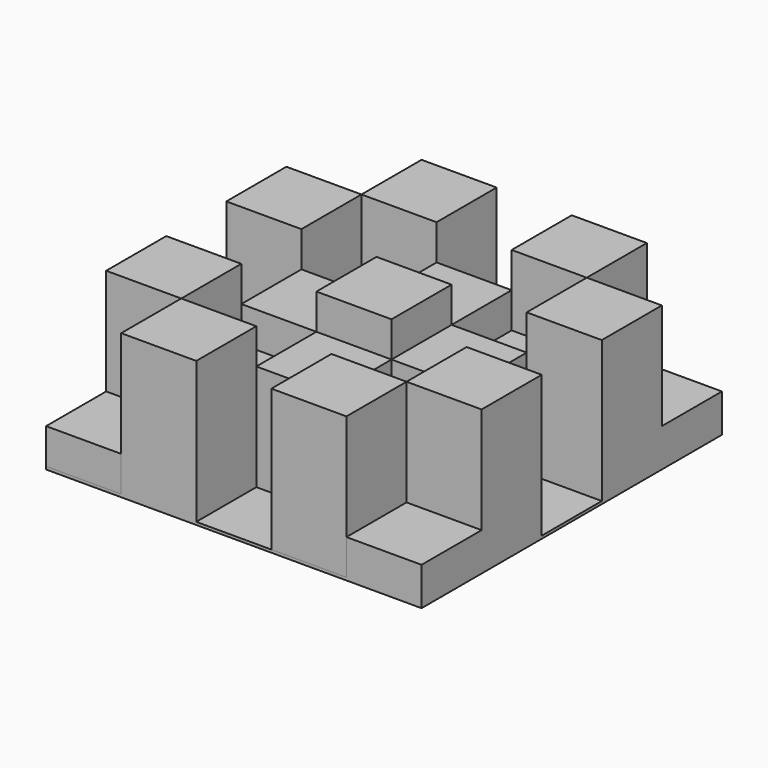
from build123d import *

# Parameters (mm, degrees)
F0_W     = 26.9276529551
F0_H     = 26.9276529551
F1_DEPTH = 38.1
F2_DEPTH = 25.4
F3_DEPTH = 12.7
F4_DEPTH = 50.8
F8_DEPTH = 1


with BuildPart() as f1:
    # F0 (on Top) → F1 (new body)
    with BuildSketch(Plane.XY):
        with Locations((-26.9276529551, 0)):
            Rectangle(F0_W, F0_H)
    extrude(amount=F1_DEPTH)



with BuildPart() as f1b:
    # F0 (on Top) → F1, piece 2 (new body)
    with BuildSketch(Plane.XY):
        with Locations((0, 26.9276529551)):
            Rectangle(F0_W, F0_H)
    extrude(amount=F1_DEPTH)


with BuildPart() as f1c:
    # F0 (on Top) → F1, piece 3 (new body)
    with BuildSketch(Plane.XY):
        with Locations((26.9276529551, 0)):
            Rectangle(F0_W, F0_H)
    extrude(amount=F1_DEPTH)


with BuildPart() as f1d:
    # F0 (on Top) → F1, piece 4 (new body)
    with BuildSketch(Plane.XY):
        with Locations((0, -26.9276529551)):
            Rectangle(F0_W, F0_H)
    extrude(amount=F1_DEPTH)


with BuildPart() as f1_1:
    add(f1.part)

    add(f1b.part)  # F2 merges F1b

    add(f1c.part)  # F2 merges F1c

    add(f1d.part)  # F2 merges F1d
    # F0 (on Top) → F2 (join)
    with BuildSketch(Plane.XY):
        with Locations((-26.9276529551, -26.9276529551)):
            Rectangle(F0_W, F0_H)
        with Locations((-26.9276529551, 26.9276529551)):
            Rectangle(F0_W, F0_H)
        with Locations((26.9276529551, 26.9276529551)):
            Rectangle(F0_W, F0_H)
        with Locations((26.9276529551, -26.9276529551)):
            Rectangle(F0_W, F0_H)
    extrude(amount=F2_DEPTH)

    # F0 (on Top) → F4, piece 9 (join)
    with BuildSketch(Plane.XY):
        Rectangle(F0_W, F0_H)
    extrude(amount=F4_DEPTH)


with BuildPart() as f3:
    # F0 (on Top) → F3 (new body)
    with BuildSketch(Plane.XY):
        with Locations((-53.8553059101, 53.8553059101)):
            Rectangle(F0_W, F0_H)
    extrude(amount=F3_DEPTH)

    # F0 (on Top) → F4 (join)
    with BuildSketch(Plane.XY):
        with Locations((-53.8553059101, 26.9276529551)):
            Rectangle(F0_W, F0_H)
    extrude(amount=F4_DEPTH)


with BuildPart() as f3b:
    # F0 (on Top) → F3, piece 2 (new body)
    with BuildSketch(Plane.XY):
        with Locations((-53.8553059101, -53.8553059101)):
            Rectangle(F0_W, F0_H)
    extrude(amount=F3_DEPTH)

    # F0 (on Top) → F4, piece 8 (join)
    with BuildSketch(Plane.XY):
        with Locations((-53.8553059101, -26.9276529551)):
            Rectangle(F0_W, F0_H)
    extrude(amount=F4_DEPTH)

    # F5: union 


with BuildPart() as f3c:
    # F0 (on Top) → F3, piece 3 (new body)
    with BuildSketch(Plane.XY):
        with Locations((53.8553059101, 53.8553059101)):
            Rectangle(F0_W, F0_H)
    extrude(amount=F3_DEPTH)

    # F0 (on Top) → F4, piece 4 (join)
    with BuildSketch(Plane.XY):
        with Locations((53.8553059101, 26.9276529551)):
            Rectangle(F0_W, F0_H)
    extrude(amount=F4_DEPTH)

    # F6: union 



with BuildPart() as f3d:
    # F0 (on Top) → F3, piece 4 (new body)
    with BuildSketch(Plane.XY):
        with Locations((53.8553059101, -53.8553059101)):
            Rectangle(F0_W, F0_H)
    extrude(amount=F3_DEPTH)

    # F0 (on Top) → F4, piece 5 (join)
    with BuildSketch(Plane.XY):
        with Locations((53.8553059101, -26.9276529551)):
            Rectangle(F0_W, F0_H)
    extrude(amount=F4_DEPTH)


with BuildPart() as f4:
    # F0 (on Top) → F4, piece 2 (new body)
    with BuildSketch(Plane.XY):
        with Locations((-26.9276529551, 53.8553059101)):
            Rectangle(F0_W, F0_H)
    extrude(amount=F4_DEPTH)


with BuildPart() as f4b:
    # F0 (on Top) → F4, piece 3 (new body)
    with BuildSketch(Plane.XY):
        with Locations((26.9276529551, 53.8553059101)):
            Rectangle(F0_W, F0_H)
    extrude(amount=F4_DEPTH)


with BuildPart() as f4c:
    # F0 (on Top) → F4, piece 6 (new body)
    with BuildSketch(Plane.XY):
        with Locations((26.9276529551, -53.8553059101)):
            Rectangle(F0_W, F0_H)
    extrude(amount=F4_DEPTH)


with BuildPart() as f4d:
    # F0 (on Top) → F4, piece 7 (new body)
    with BuildSketch(Plane.XY):
        with Locations((-26.9276529551, -53.8553059101)):
            Rectangle(F0_W, F0_H)
    extrude(amount=F4_DEPTH)


with BuildPart() as f3c_1:
    add(f3c.part)

    add(f3d.part)  # F8 merges F3d

    add(f4d.part)  # F8 merges F4d
    # F7 (on face) → F8 (join)
    with BuildSketch(Plane(origin=(0, 0, 0), x_dir=(1, 0, 0), z_dir=(0, 0, -1))):
        Polygon((-67.3191323876, -67.3191323876), (67.3191323876, -67.3191323876), (67.3191323876, -13.4638264775), (67.3191323876, 67.3191323876), (-67.3191323876, 67.3191323876), (-67.3191323876, 13.4638264775), align=None)
    extrude(amount=F8_DEPTH)


solid = Compound([f1_1.part, f3.part, f3b.part, f4.part, f4b.part, f4c.part, f3c_1.part])
